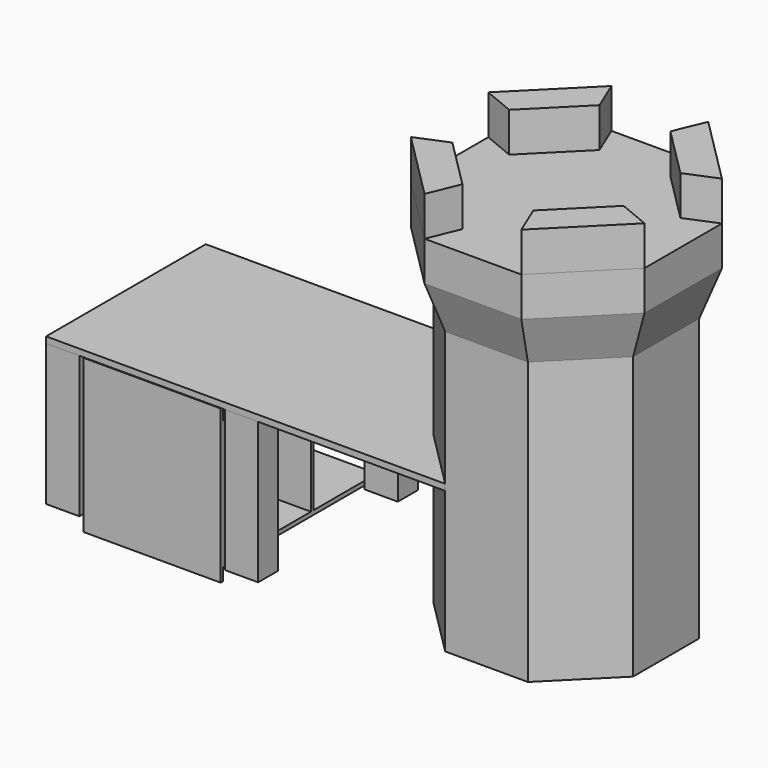
from build123d import *

# Parameters (mm, degrees)
F3_DEPTH      = 38.1
F4_W          = 203.2
F4_H          = 152.4
F5_DEPTH      = 863.6
F8_DEPTH      = 863.6
F8_DEPTH_BACK = 857.0384116704
F10_DEPTH     = 285.9615883296
F10_TAPER     = -20
F12_DEPTH     = 241.3
F14_DEPTH     = 241.3
F15_W         = 38.1
F15_H         = 812.8
F16_DEPTH     = 88.9
F18_W         = 838.2
F18_H         = 1174.75
F19_DEPTH     = 25.4
F21_W         = 838.2
F21_H         = 936.625
F22_DEPTH     = 19.05
F23_W         = 19.05
F23_H         = 165.1
F24_DEPTH     = 762
F25_W         = 19.05
F25_H         = 485.775
F25_H_2       = 19.05
F25_W_2       = 409.575
F26_DEPTH     = 762


with BuildPart() as f3:
    # F2 (on Top) → F3 (new body)
    with BuildSketch(Plane.XY):
        Polygon((-1219.2, 609.6), (-1219.2, -609.6), (1219.2, -609.6), (862.1045876226, -252.5045876226), (862.1045876226, 252.5045876226), (1219.2, 609.6), align=None)
    extrude(amount=F3_DEPTH)


with BuildPart() as f5:
    # F4 (on Top) → F5 (new body, through all)
    with BuildSketch(Plane.XY):
        with Locations((-1117.6, 533.4)):
            Rectangle(F4_W, F4_H)
    extrude(amount=-F5_DEPTH)


with BuildPart() as f5b:
    # F4 (on Top) → F5, piece 2 (new body, through all)
    with BuildSketch(Plane.XY):
        with Locations((-1117.6, -533.4)):
            Rectangle(F4_W, F4_H)
    extrude(amount=-F5_DEPTH)


with BuildPart() as f5c:
    # F4 (on Top) → F5, piece 3 (new body, through all)
    with BuildSketch(Plane.XY):
        with Locations((-25.4, 533.4)):
            Rectangle(F4_W, F4_H)
    extrude(amount=-F5_DEPTH)


with BuildPart() as f5d:
    # F4 (on Top) → F5, piece 4 (new body, through all)
    with BuildSketch(Plane.XY):
        with Locations((-25.4, -533.4)):
            Rectangle(F4_W, F4_H)
    extrude(amount=-F5_DEPTH)


with BuildPart() as f8:
    # F7 (on Top) → F8 (new body, two sides)
    with BuildSketch(Plane.XY) as f8_sk:
        Polygon((1219.2, -609.6), (1724.2091752453, -609.6), (2081.3045876226, -252.5045876226), (2081.3045876226, 252.5045876226), (1724.2091752453, 609.6), (1219.2, 609.6), (862.1045876226, 252.5045876226), (862.1045876226, -252.5045876226), align=None)
    extrude(amount=-F8_DEPTH)
    extrude(f8_sk.sketch, amount=F8_DEPTH_BACK)


with BuildPart() as f10:
    # F9 (on face) → F10 (new body, through all)
    with BuildSketch(Plane.XY.offset(857.0384116704)):
        Polygon((862.1045876226, 252.5045876226), (862.1045876226, -252.5045876226), (1219.2, -609.6), (1724.2091752453, -609.6), (2081.3045876226, -252.5045876226), (2081.3045876226, 252.5045876226), (1724.2091752453, 609.6), (1219.2, 609.6), align=None)
    extrude(amount=F10_DEPTH, taper=F10_TAPER)


with BuildPart() as f12:
    # F11 (on face) → F12 (new body, through all)
    with BuildSketch(Plane.XY.offset(1143)):
        Polygon((1767.3211467451, 713.6815062955), (1176.0880285002, 713.6815062955), (758.0230813272, 295.6165591224), (758.0230813272, -295.6165591224), (1176.0880285002, -713.6815062955), (1767.3211467451, -713.6815062955), (2185.3860939181, -295.6165591224), (2185.3860939181, 295.6165591224), align=None)
    extrude(amount=F12_DEPTH)


with BuildPart() as f14:
    # F13 (on face) → F14 (new body, through all)
    with BuildSketch(Plane.XY.offset(1384.3)):
        Polygon((1254.9957121323, 523.1815062955), (1176.0880285002, 713.6815062955), (758.0230813272, 295.6165591224), (948.5230813272, 216.7088754904), align=None)
    extrude(amount=F14_DEPTH)


with BuildPart() as f14b:
    # F13 (on face) → F14, piece 2 (new body, through all)
    with BuildSketch(Plane.XY.offset(1384.3)):
        Polygon((2185.3860939181, 295.6165591224), (1767.3211467451, 713.6815062955), (1688.413463113, 523.1815062955), (1994.8860939181, 216.7088754904), align=None)
    extrude(amount=F14_DEPTH)


with BuildPart() as f14c:
    # F13 (on face) → F14, piece 3 (new body, through all)
    with BuildSketch(Plane.XY.offset(1384.3)):
        Polygon((1767.3211467451, -713.6815062955), (2185.3860939181, -295.6165591224), (1994.8860939181, -216.7088754904), (1688.413463113, -523.1815062955), align=None)
    extrude(amount=F14_DEPTH)


with BuildPart() as f14d:
    # F13 (on face) → F14, piece 4 (new body, through all)
    with BuildSketch(Plane.XY.offset(1384.3)):
        Polygon((948.5230813272, -216.7088754904), (758.0230813272, -295.6165591224), (1176.0880285002, -713.6815062955), (1254.9957121323, -523.1815062955), align=None)
    extrude(amount=F14_DEPTH)


with BuildPart() as f16:
    # F15 (on Top) → F16 (new body)
    with BuildSketch(Plane.XY):
        with Locations((-146.05, 0)):
            Rectangle(F15_W, F15_H)
        Polygon((-977.9, -406.4), (-1016, -406.4), (-1016, -457.2), (-127, -457.2), (-127, -406.4), (-165.1, -406.4), align=None)
        with Locations((-996.95, 0)):
            Rectangle(F15_W, F15_H)
        Polygon((-127, 457.2), (-1016, 457.2), (-1016, 406.4), (-977.9, 406.4), (-165.1, 406.4), (-127, 406.4), align=None)
    extrude(amount=-F16_DEPTH)


with BuildPart() as f19:
    # F18 (on plane+point) → F19 (new body)
    with BuildSketch(Plane.XY.offset(-863.6)):
        with Locations((-571.5, -3.175)):
            Rectangle(F18_W, F18_H)
    extrude(amount=F19_DEPTH)


with BuildPart() as f22:
    # F21 (on plane+point) → F22 (new body, through all)
    with BuildSketch(Plane.XZ.offset(590.55)):
        with Locations((-571.5, -471.4875)):
            Rectangle(F21_W, F21_H)
    extrude(amount=F22_DEPTH)


with BuildPart() as f24:
    # F23 (on face) → F24 (new body)
    with BuildSketch(Plane.XY.offset(-838.2)):
        Polygon((-152.4, -406.4), (-990.6, -406.4), (-990.6, -425.45), (-971.55, -425.45), (-171.45, -425.45), (-152.4, -425.45), align=None)
        with Locations((-981.075, -508)):
            Rectangle(F23_W, F23_H)
        with Locations((-161.925, -508)):
            Rectangle(F23_W, F23_H)
    extrude(amount=F24_DEPTH)


with BuildPart() as f26:
    # F25 (on face) → F26 (new body)
    with BuildSketch(Plane.XY.offset(-838.2)):
        with Locations((-571.5, 341.3125)):
            Rectangle(F25_W, F25_H)
        with Locations((-571.5, 88.9)):
            Rectangle(F25_W, F25_H_2)
        with Locations((-785.8125, 88.9)):
            Rectangle(F25_W_2, F25_H_2)
        with Locations((-357.1875, 88.9)):
            Rectangle(F25_W_2, F25_H_2)
        with Locations((-571.5, -163.5125)):
            Rectangle(F25_W, F25_H)
    extrude(amount=F26_DEPTH)


solid = Compound([f3.part, f5.part, f5b.part, f5c.part, f5d.part, f8.part, f10.part, f12.part, f14.part, f14b.part, f14c.part, f14d.part, f16.part, f19.part, f22.part, f24.part, f26.part])
